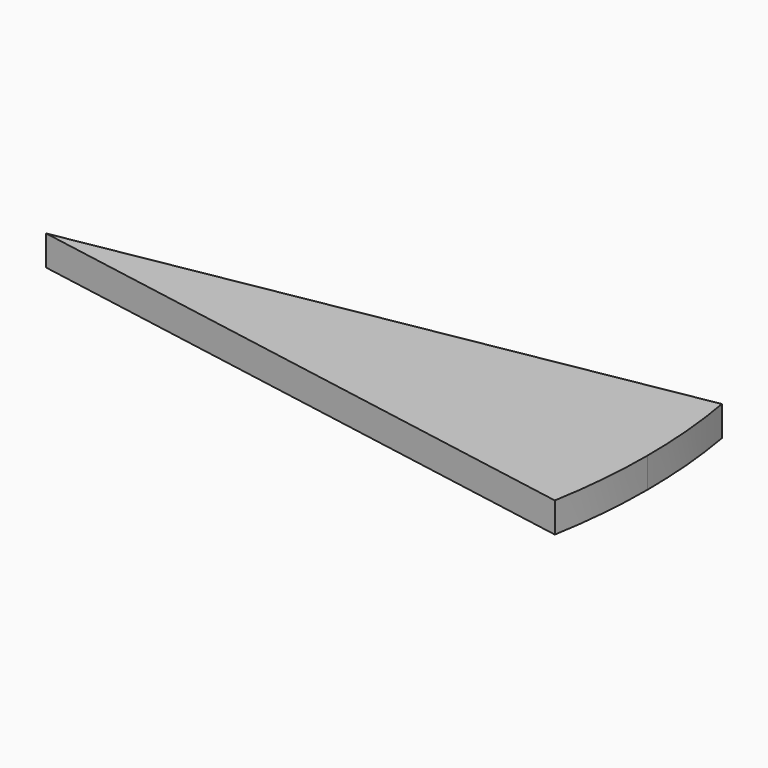
from build123d import *

# Parameters (mm, degrees)
F1_DEPTH = 5


# Not quite as in the source:
# - a feature of the source that left no trace in its solid (it failed there, or was rolled back) is left out


with BuildPart() as f1:
    # F0 (on Top) → F1 (new body)
    with BuildSketch(Plane.XY):
        with BuildLine():
            Line((0, 0), (98.4807753012, -17.3648177667))
            ThreePointArc((98.4807753012, -17.3648177667), (99.6194698092, -8.7155742748), (100, 0))
            Line((100, 0), (0, 0))
        make_face()
        with BuildLine():
            Line((0, 0), (100, 0))
            ThreePointArc((100, 0), (99.6194698092, 8.7155742748), (98.4807753012, 17.3648177667))
            Line((98.4807753012, 17.3648177667), (0, 0))
        make_face()
    extrude(amount=F1_DEPTH)


solid = f1.part
